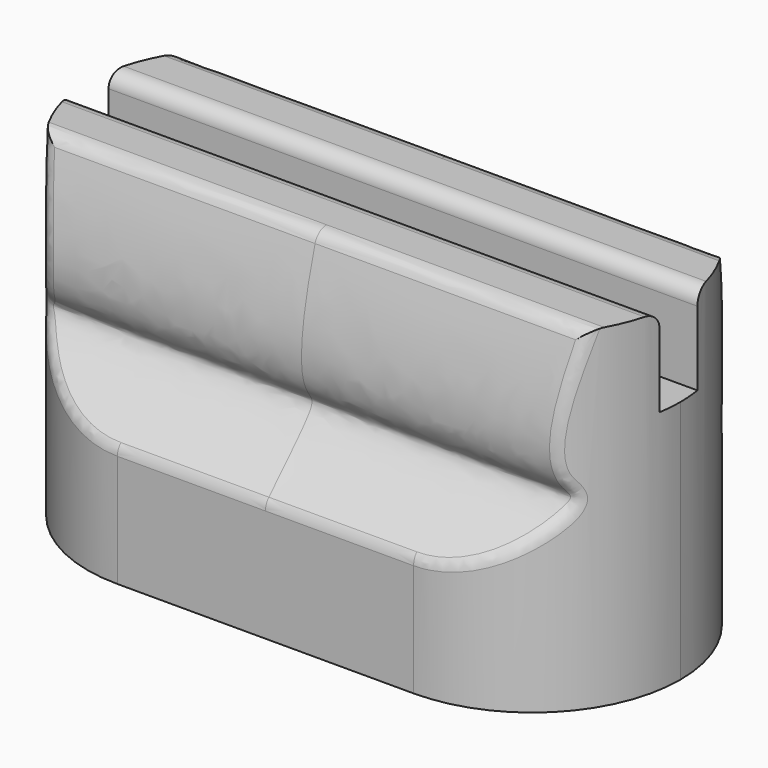
from build123d import *

# Parameters (mm, degrees)
F1_DEPTH = 10
F3_DEPTH = 11.2510001
F5_D     = 3
F5_DEPTH = 7
F5_TIP   = 0.9012909285
F6_R     = 0.5


with BuildPart() as f1:
    # F0 (on Right) → F1 (new body, symmetric)
    with BuildSketch(Plane.YZ):
        with BuildLine():
            add(Edge.make_bspline(
                [(2.8, 11.25), (5, 4), (0.8, 8.25), (5, 4)],
                knots=[0, 0, 0, 0, 7.5764437568, 7.5764437568, 7.5764437568, 7.5764437568], degree=3))
            Line((2.8, 11.25), (0.8, 11.25))
            Line((0.8, 11.25), (0.8, 8.25))
            Line((0.8, 8.25), (-0.8, 8.25))
            Line((-0.8, 8.25), (-0.8, 11.25))
            Line((-0.8, 11.25), (-2.8, 11.25))
            add(Edge.make_bspline(
                [(-2.8, 11.25), (-5, 4), (-0.8, 8.25), (-5, 4)],
                knots=[0, 0, 0, 0, 7.5764437568, 7.5764437568, 7.5764437568, 7.5764437568], degree=3))
            Line((-5, 4), (-5, 0))
            Line((-5, 0), (5, 0))
            Line((5, 0), (5, 4))
        make_face()
    extrude(amount=F1_DEPTH, both=True)

    # F2 (on face) → F3 (intersect, through all)
    with BuildSketch(Plane(origin=(0, 0, 0), x_dir=(1, 0, 0), z_dir=(0, 0, -1))):
        with BuildLine():
            Line((5, 5), (-5, 5))
            ThreePointArc((-5, 5), (-8.5355339059, 3.5355339059), (-10, 0))
            ThreePointArc((-10, 0), (-8.5355339059, -3.5355339059), (-5, -5))
            Line((-5, -5), (5, -5))
            ThreePointArc((5, -5), (8.5355339059, -3.5355339059), (10, 0))
            ThreePointArc((10, 0), (8.5355339059, 3.5355339059), (5, 5))
        make_face()
    extrude(amount=-F3_DEPTH, mode=Mode.INTERSECT)

    # F5
    with Locations(Plane(origin=(0, 0, 0), x_dir=(1, 0, 0), z_dir=(0, 0, -1))):
        with Locations((0, 0)):
            Hole(F5_D / 2, depth=F5_DEPTH)
            with Locations((0, 0, -(F5_DEPTH + F5_TIP / 2))):  # 118° drill point
                Cone(0, F5_D / 2, F5_TIP, mode=Mode.SUBTRACT)

    # F6
    f6_edges = [f1.edges().sort_by_distance(p)[0] for p in [
        (-4.571232, -2.8, 11.25),
        (4.571232, -2.8, 11.25),
        (0, -0.8, 11.25),
        (0, 0.8, 11.25),
        (-4.571232, 2.8, 11.25),
        (4.571232, 2.8, 11.25),
        (-2.5, 5, 4),
        (2.5, 5, 4),
        (0, -3.442785, 7.233073),
        (-2.5, -5, 4),
        (-8.971055, -3.03821, 6.240026),
        (2.5, -5, 4),
        (-8.945777, 3.070968, 6.370826),
        (8.945777, 3.070968, 6.370826),
        (8.945777, -3.070968, 6.370826),
    ]]
    fillet(f6_edges, radius=F6_R)


solid = f1.part
